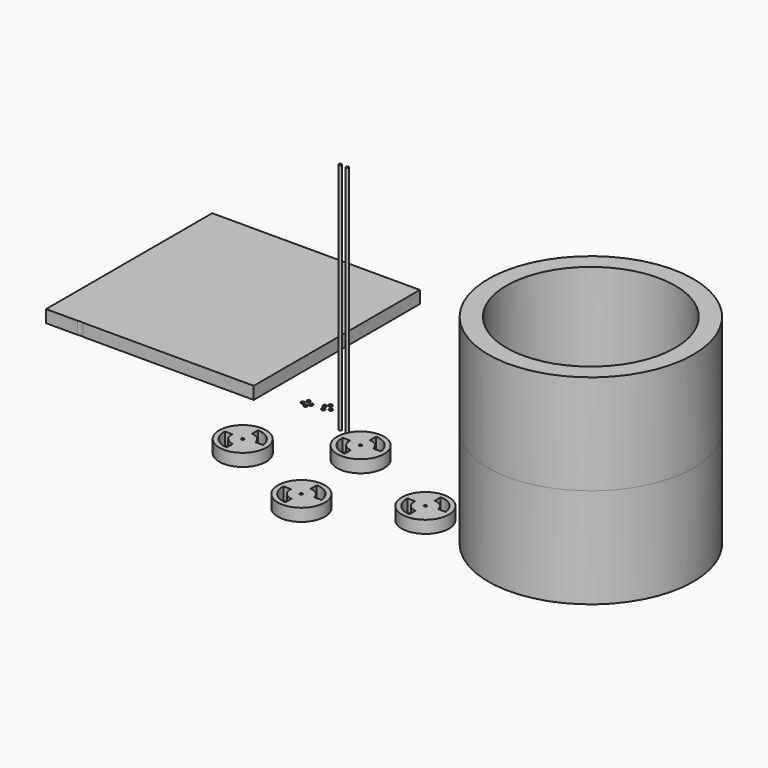
from build123d import *

# Parameters (mm, degrees)
F1_DEPTH = 6.096
F2_R     = 50.165
F2_R_2   = 41.275
F3_DEPTH = 48.895
F4_R     = 11.4975103392
F4_R_2   = 0.6991975049
F5_DEPTH = 6.096
F6_R     = 0.6858
F7_DEPTH = 114.3
F8_R     = 0.8255
F8_R_2   = 0.6985
F9_DEPTH = 0.254


# Not quite as in the source:
# - a feature names something its author has since deleted; it is built from what else it names
# - the program builds the solid bodies; features that only make, move or delete a surface that nothing else refers to are left out


with BuildPart() as f1:
    # F0 (on Top) → F1 (new body)
    with BuildSketch(Plane.XY):
        with BuildLine():
            Line((-104.046491341, 59.8414842989), (-104.046491341, -41.7585157011))
            Line((-104.046491341, -41.7585157011), (-88.5665284773, -41.7585157011))
            ThreePointArc((-88.5665284773, -41.7585157011), (-87.2272327542, -41.6239274504), (-85.8879370312, -41.7585157011))
            Line((-85.8879370312, -41.7585157011), (-2.446491341, -41.7585157011))
            Line((-2.446491341, -41.7585157011), (-2.446491341, 59.8414842989))
            Line((-2.446491341, 59.8414842989), (-104.046491341, 59.8414842989))
        make_face()
    extrude(amount=F1_DEPTH)


with BuildPart() as f3:
    # F2 (on Top) → F3 (new body, symmetric)
    with BuildSketch(Plane.XY):
        with Locations((113.8069406152, 19.1121064126)):
            Circle(F2_R)
        with Locations((113.8069406152, 19.1121064126)):
            Circle(F2_R_2, mode=Mode.SUBTRACT)
    extrude(amount=-F3_DEPTH, both=True)


with BuildPart() as f5:
    # F4 (on Top) → F5 (new body)
    with BuildSketch(Plane.XY):
        with Locations((60.2071579216, -54.7079068924)):
            Circle(F4_R)
        with BuildLine():
            ThreePointArc((54.6990466325, -54.1260507265), (55.9541472068, -58.2561101603), (59.7923801425, -60.2311130233))
            Line((59.7923801425, -60.2311130233), (59.7923801425, -63.9349583017))
            ThreePointArc((59.7923801425, -63.9349583017), (53.3331937637, -60.8771155186), (50.989134179, -54.1260507265))
            Line((50.989134179, -54.1260507265), (54.6990466325, -54.1260507265))
        make_face(mode=Mode.SUBTRACT)
        with BuildLine():
            Line((60.4740997744, -63.9404179465), (60.4740997744, -60.2402290646))
            ThreePointArc((60.4740997744, -60.2402290646), (64.312364088, -58.4261227147), (65.7388171119, -54.4275621536))
            Line((65.7388171119, -54.4275621536), (69.4392717177, -54.4275621536))
            ThreePointArc((69.4392717177, -54.4275621536), (66.9288854443, -61.0426442529), (60.4740997744, -63.9404179465))
        make_face(mode=Mode.SUBTRACT)
        with Locations((60.2071579216, -54.7079068924)):
            Circle(F4_R_2, mode=Mode.SUBTRACT)
        with BuildLine():
            ThreePointArc((51.0549450288, -53.4639143353), (53.7753044223, -48.0790473464), (59.239770012, -45.5223378328))
            Line((59.239770012, -45.5223378328), (59.239770012, -49.2542835829))
            ThreePointArc((59.239770012, -49.2542835829), (56.3917407696, -50.6928803014), (54.8099059275, -53.4639143353))
            Line((54.8099059275, -53.4639143353), (51.0549450288, -53.4639143353))
        make_face(mode=Mode.SUBTRACT)
        with BuildLine():
            Line((60.3225569605, -49.1703506054), (60.3225569605, -45.4722584918))
            ThreePointArc((60.3225569605, -45.4722584918), (66.4389794286, -47.8906553185), (69.3953691609, -53.7659448238))
            Line((69.3953691609, -53.7659448238), (65.6652302948, -53.7659448238))
            ThreePointArc((65.6652302948, -53.7659448238), (63.8190504242, -50.5088499603), (60.3225569605, -49.1703506054))
        make_face(mode=Mode.SUBTRACT)
        with BuildLine():
            ThreePointArc((65.7388171119, -54.4275621536), (64.312364088, -58.4261227147), (60.4740997744, -60.2402290646))
            Line((60.4740997744, -60.2402290646), (60.4740997744, -63.9404179465))
            ThreePointArc((60.4740997744, -63.9404179465), (66.9288854443, -61.0426442529), (69.4392717177, -54.4275621536))
            Line((69.4392717177, -54.4275621536), (65.7388171119, -54.4275621536))
        make_face()
        with BuildLine():
            Line((59.239770012, -49.2542835829), (59.239770012, -45.5223378328))
            ThreePointArc((59.239770012, -45.5223378328), (53.7753044223, -48.0790473464), (51.0549450288, -53.4639143353))
            Line((51.0549450288, -53.4639143353), (54.8099059275, -53.4639143353))
            ThreePointArc((54.8099059275, -53.4639143353), (56.3917407696, -50.6928803014), (59.239770012, -49.2542835829))
        make_face()
    extrude(amount=F5_DEPTH)


with BuildPart() as f5b:
    # F4 (on Top) → F5, piece 2 (new body)
    with BuildSketch(Plane.XY):
        with Locations((110.8582236975, -78.3851350165)):
            Circle(F4_R)
        with BuildLine():
            Line((101.6401999549, -77.8032788507), (105.3501124085, -77.8032788507))
            ThreePointArc((105.3501124085, -77.8032788507), (106.6052129827, -81.9333382844), (110.4434459184, -83.9083411474))
            Line((110.4434459184, -83.9083411474), (110.4434459184, -87.6121864259))
            ThreePointArc((110.4434459184, -87.6121864259), (103.9842595396, -84.5543436427), (101.6401999549, -77.8032788507))
        make_face(mode=Mode.SUBTRACT)
        with BuildLine():
            ThreePointArc((111.1251655504, -83.9174571887), (114.963429864, -82.1033508388), (116.3898828878, -78.1047902777))
            Line((116.3898828878, -78.1047902777), (120.0903374936, -78.1047902777))
            ThreePointArc((120.0903374936, -78.1047902777), (117.5799512202, -84.7198723771), (111.1251655504, -87.6176460706))
            Line((111.1251655504, -87.6176460706), (111.1251655504, -83.9174571887))
        make_face(mode=Mode.SUBTRACT)
        with Locations((110.8582236975, -78.3851350165)):
            Circle(F4_R_2, mode=Mode.SUBTRACT)
        with BuildLine():
            ThreePointArc((101.7060108047, -77.1411424594), (104.4263701982, -71.7562754705), (109.8908357879, -69.1995659569))
            Line((109.8908357879, -69.1995659569), (109.8908357879, -72.931511707))
            ThreePointArc((109.8908357879, -72.931511707), (107.0428065455, -74.3701084256), (105.4609717034, -77.1411424594))
            Line((105.4609717034, -77.1411424594), (101.7060108047, -77.1411424594))
        make_face(mode=Mode.SUBTRACT)
        with BuildLine():
            Line((110.9736227364, -72.8475787295), (110.9736227364, -69.149486616))
            ThreePointArc((110.9736227364, -69.149486616), (117.0900452046, -71.5678834427), (120.0464349368, -77.443172948))
            Line((120.0464349368, -77.443172948), (116.3162960707, -77.443172948))
            ThreePointArc((116.3162960707, -77.443172948), (114.4701162002, -74.1860780844), (110.9736227364, -72.8475787295))
        make_face(mode=Mode.SUBTRACT)
        with BuildLine():
            Line((120.0903374936, -78.1047902777), (116.3898828878, -78.1047902777))
            ThreePointArc((116.3898828878, -78.1047902777), (114.963429864, -82.1033508388), (111.1251655504, -83.9174571887))
            Line((111.1251655504, -83.9174571887), (111.1251655504, -87.6176460706))
            ThreePointArc((111.1251655504, -87.6176460706), (117.5799512202, -84.7198723771), (120.0903374936, -78.1047902777))
        make_face()
        with BuildLine():
            Line((109.8908357879, -72.931511707), (109.8908357879, -69.1995659569))
            ThreePointArc((109.8908357879, -69.1995659569), (104.4263701982, -71.7562754705), (101.7060108047, -77.1411424594))
            Line((101.7060108047, -77.1411424594), (105.4609717034, -77.1411424594))
            ThreePointArc((105.4609717034, -77.1411424594), (107.0428065455, -74.3701084256), (109.8908357879, -72.931511707))
        make_face()
    extrude(amount=F5_DEPTH)


with BuildPart() as f5c:
    # F4 (on Top) → F5, piece 3 (new body)
    with BuildSketch(Plane.XY):
        with Locations((21.7524592936, -78.7456388093)):
            Circle(F4_R)
        with BuildLine():
            Line((12.534435551, -78.1637826434), (16.2443480046, -78.1637826434))
            ThreePointArc((16.2443480046, -78.1637826434), (17.4994485788, -82.2938420771), (21.3376815145, -84.2688449401))
            Line((21.3376815145, -84.2688449401), (21.3376815145, -87.9726902186))
            ThreePointArc((21.3376815145, -87.9726902186), (14.8784951357, -84.9148474354), (12.534435551, -78.1637826434))
        make_face(mode=Mode.SUBTRACT)
        with Locations((21.7524592936, -78.7456388093)):
            Circle(F4_R_2, mode=Mode.SUBTRACT)
        with BuildLine():
            ThreePointArc((30.9845730897, -78.4652940705), (28.4741868163, -85.0803761698), (22.0194011464, -87.9781498634))
            Line((22.0194011464, -87.9781498634), (22.0194011464, -84.2779609815))
            ThreePointArc((22.0194011464, -84.2779609815), (25.85766546, -82.4638546316), (27.2841184839, -78.4652940705))
            Line((27.2841184839, -78.4652940705), (30.9845730897, -78.4652940705))
        make_face(mode=Mode.SUBTRACT)
        with BuildLine():
            ThreePointArc((12.6002464008, -77.5016462522), (15.3206057943, -72.1167792633), (20.785071384, -69.5600697497))
            Line((20.785071384, -69.5600697497), (20.785071384, -73.2920154997))
            ThreePointArc((20.785071384, -73.2920154997), (17.9370421416, -74.7306122183), (16.3552072995, -77.5016462522))
            Line((16.3552072995, -77.5016462522), (12.6002464008, -77.5016462522))
        make_face(mode=Mode.SUBTRACT)
        with BuildLine():
            ThreePointArc((27.2105316668, -77.8036767407), (25.3643517962, -74.5465818771), (21.8678583325, -73.2080825223))
            Line((21.8678583325, -73.2080825223), (21.8678583325, -69.5099904087))
            ThreePointArc((21.8678583325, -69.5099904087), (27.9842808006, -71.9283872354), (30.9406705329, -77.8036767407))
            Line((30.9406705329, -77.8036767407), (27.2105316668, -77.8036767407))
        make_face(mode=Mode.SUBTRACT)
        with BuildLine():
            Line((22.0194011464, -84.2779609815), (22.0194011464, -87.9781498634))
            ThreePointArc((22.0194011464, -87.9781498634), (28.4741868163, -85.0803761698), (30.9845730897, -78.4652940705))
            Line((30.9845730897, -78.4652940705), (27.2841184839, -78.4652940705))
            ThreePointArc((27.2841184839, -78.4652940705), (25.85766546, -82.4638546316), (22.0194011464, -84.2779609815))
        make_face()
        with BuildLine():
            Line((20.785071384, -73.2920154997), (20.785071384, -69.5600697497))
            ThreePointArc((20.785071384, -69.5600697497), (15.3206057943, -72.1167792633), (12.6002464008, -77.5016462522))
            Line((12.6002464008, -77.5016462522), (16.3552072995, -77.5016462522))
            ThreePointArc((16.3552072995, -77.5016462522), (17.9370421416, -74.7306122183), (20.785071384, -73.2920154997))
        make_face()
    extrude(amount=F5_DEPTH)


with BuildPart() as f5d:
    # F4 (on Top) → F5, piece 4 (new body)
    with BuildSketch(Plane.XY):
        with Locations((67.6437759012, -100.240712843)):
            Circle(F4_R)
        with BuildLine():
            ThreePointArc((62.1356646121, -99.6588566772), (63.3907651864, -103.7889161109), (67.2289981221, -105.7639189739))
            Line((67.2289981221, -105.7639189739), (67.2289981221, -109.4677642524))
            ThreePointArc((67.2289981221, -109.4677642524), (60.7698117433, -106.4099214692), (58.4257521586, -99.6588566772))
            Line((58.4257521586, -99.6588566772), (62.1356646121, -99.6588566772))
        make_face(mode=Mode.SUBTRACT)
        with BuildLine():
            ThreePointArc((58.4915630084, -98.9967202859), (61.2119224019, -93.611853297), (66.6763879916, -91.0551437834))
            Line((66.6763879916, -91.0551437834), (66.6763879916, -94.7870895335))
            ThreePointArc((66.6763879916, -94.7870895335), (63.8283587492, -96.2256862521), (62.2465239071, -98.9967202859))
            Line((62.2465239071, -98.9967202859), (58.4915630084, -98.9967202859))
        make_face(mode=Mode.SUBTRACT)
        with BuildLine():
            ThreePointArc((67.910717754, -105.7730350152), (71.7489820676, -103.9589286653), (73.1754350915, -99.9603681042))
            Line((73.1754350915, -99.9603681042), (76.8758896973, -99.9603681042))
            ThreePointArc((76.8758896973, -99.9603681042), (74.3655034239, -106.5754502036), (67.910717754, -109.4732238971))
            Line((67.910717754, -109.4732238971), (67.910717754, -105.7730350152))
        make_face(mode=Mode.SUBTRACT)
        with Locations((67.6437759012, -100.240712843)):
            Circle(F4_R_2, mode=Mode.SUBTRACT)
        with BuildLine():
            Line((76.8319871405, -99.2987507745), (73.1018482744, -99.2987507745))
            ThreePointArc((73.1018482744, -99.2987507745), (71.2556684038, -96.0416559109), (67.7591749401, -94.703156556))
            Line((67.7591749401, -94.703156556), (67.7591749401, -91.0050644425))
            ThreePointArc((67.7591749401, -91.0050644425), (73.8755974082, -93.4234612692), (76.8319871405, -99.2987507745))
        make_face(mode=Mode.SUBTRACT)
        with BuildLine():
            Line((76.8758896973, -99.9603681042), (73.1754350915, -99.9603681042))
            ThreePointArc((73.1754350915, -99.9603681042), (71.7489820676, -103.9589286653), (67.910717754, -105.7730350152))
            Line((67.910717754, -105.7730350152), (67.910717754, -109.4732238971))
            ThreePointArc((67.910717754, -109.4732238971), (74.3655034239, -106.5754502036), (76.8758896973, -99.9603681042))
        make_face()
        with BuildLine():
            Line((66.6763879916, -94.7870895335), (66.6763879916, -91.0551437834))
            ThreePointArc((66.6763879916, -91.0551437834), (61.2119224019, -93.611853297), (58.4915630084, -98.9967202859))
            Line((58.4915630084, -98.9967202859), (62.2465239071, -98.9967202859))
            ThreePointArc((62.2465239071, -98.9967202859), (63.8283587492, -96.2256862521), (66.6763879916, -94.7870895335))
        make_face()
    extrude(amount=F5_DEPTH)


with BuildPart() as f7:
    # F6 (on Top) → F7 (new body)
    with BuildSketch(Plane.XY):
        with Locations((38.8235077262, -40.3998494148)):
            Circle(F6_R)
    extrude(amount=F7_DEPTH)


with BuildPart() as f7b:
    # F6 (on Top) → F7, piece 2 (new body)
    with BuildSketch(Plane.XY):
        with Locations((42.3253141344, -40.4072664678)):
            Circle(F6_R)
    extrude(amount=F7_DEPTH)


with BuildPart() as f9:
    # F8 (on Top) → F9 (new body)
    with BuildSketch(Plane.XY):
        with Locations((14.7318905219, -29.7516137362)):
            Circle(F8_R)
        with Locations((14.7318905219, -29.7516137362)):
            Circle(F8_R_2, mode=Mode.SUBTRACT)
    extrude(amount=F9_DEPTH)


with BuildPart() as f9b:
    # F8 (on Top) → F9, piece 2 (new body)
    with BuildSketch(Plane.XY):
        with Locations((17.2707214952, -31.2811471522)):
            Circle(F8_R)
        with Locations((17.2707214952, -31.2811471522)):
            Circle(F8_R_2, mode=Mode.SUBTRACT)
    extrude(amount=F9_DEPTH)


with BuildPart() as f9c:
    # F8 (on Top) → F9, piece 3 (new body)
    with BuildSketch(Plane.XY):
        with Locations((16.0888601094, -33.1985652447)):
            Circle(F8_R)
        with Locations((16.0888601094, -33.1985652447)):
            Circle(F8_R_2, mode=Mode.SUBTRACT)
    extrude(amount=F9_DEPTH)


with BuildPart() as f9d:
    # F8 (on Top) → F9, piece 4 (new body)
    with BuildSketch(Plane.XY):
        with Locations((13.6733138934, -31.9358929992)):
            Circle(F8_R)
        with Locations((13.6733138934, -31.9358929992)):
            Circle(F8_R_2, mode=Mode.SUBTRACT)
    extrude(amount=F9_DEPTH)


with BuildPart() as f9e:
    # F8 (on Top) → F9, piece 5 (new body)
    with BuildSketch(Plane.XY):
        with Locations((22.0098569989, -28.890941292)):
            Circle(F8_R)
        with Locations((22.0098569989, -28.890941292)):
            Circle(F8_R_2, mode=Mode.SUBTRACT)
    extrude(amount=F9_DEPTH)


with BuildPart() as f9f:
    # F8 (on Top) → F9, piece 6 (new body)
    with BuildSketch(Plane.XY):
        with Locations((23.5105827451, -27.1702948958)):
            Circle(F8_R)
        with Locations((23.5105827451, -27.1702948958)):
            Circle(F8_R_2, mode=Mode.SUBTRACT)
    extrude(amount=F9_DEPTH)


with BuildPart() as f9g:
    # F8 (on Top) → F9, piece 7 (new body)
    with BuildSketch(Plane.XY):
        with Locations((23.223798722, -31.2675274909)):
            Circle(F8_R)
        with Locations((23.223798722, -31.2675274909)):
            Circle(F8_R_2, mode=Mode.SUBTRACT)
    extrude(amount=F9_DEPTH)


with BuildPart() as f9h:
    # F8 (on Top) → F9, piece 8 (new body)
    with BuildSketch(Plane.XY):
        with Locations((25.6921444088, -29.8004224896)):
            Circle(F8_R)
        with Locations((25.6921444088, -29.8004224896)):
            Circle(F8_R_2, mode=Mode.SUBTRACT)
    extrude(amount=F9_DEPTH)


solid = Compound([f1.part, f3.part, f5.part, f5b.part, f5c.part, f5d.part, f7.part, f7b.part, f9.part, f9b.part, f9c.part, f9d.part, f9e.part, f9f.part, f9g.part, f9h.part])
